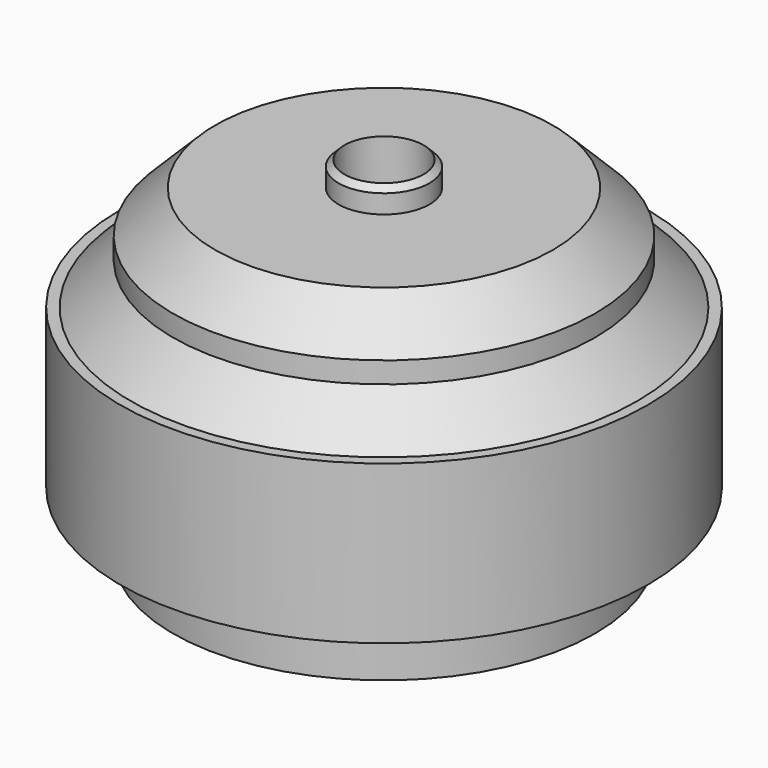
from build123d import *

# Parameters (mm, degrees)
F2_R     = 4.7625
F3_DEPTH = 9.525
F6_D     = 3.175
F6_DEPTH = 22.225
F6_START = 0.6225488
F6_TIP   = 0.9538662327
F7_SIZE  = 5.08


# Not quite as in the source:
# - a fillet or chamfer that OpenCascade refuses, or shapes differently, is made with other operations: its cross-section is extruded or revolved along the edge and cut away or added


with BuildPart() as f1:
    # F0 (on Front) → F1 (revolve)
    with BuildSketch(Plane.XZ):
        Polygon((5.470779, 56.2707707286), (0, 56.2707707286), (0, 0), (25.409779, 9.9646151066), (25.409779, 17.1938474178), (31.759779, 17.1938474178), (31.759779, 36.2438474178), (25.409779, 36.2438474178), (25.409779, 48.9438474178), (5.470779, 48.9438474178), align=None)
    revolve(axis=Axis((0, 0, 28.1353853643), (0, 0, -1)))

    # F2 (on face) → F3 (cut)
    with BuildSketch(Plane.XY.offset(56.2707707286)):
        Circle(F2_R)
    extrude(amount=-F3_DEPTH, mode=Mode.SUBTRACT)

    # F4: chamfer of 5.08 on 1 edges, made by hand

    # F4_s1 → F4_t2 (revolve, cut)
    with BuildSketch(Plane.XZ):
        Polygon((0.390779, 56.2707707286), (5.470779, 51.1907707286), (5.470779, 56.2707707286), align=None)
    revolve(axis=Axis((0, 0, 56.2707707286), (0, 0, -1)), mode=Mode.SUBTRACT)

    # F6
    # its depths count from where the whole tool has entered the part; down to there all is cleared
    with Locations(Plane(origin=(0, 0, 0), x_dir=(1, 0, 0), z_dir=(0, 0, -1)).offset(-F6_START)):
        with Locations((0, 0)):
            Hole(F6_D / 2, depth=F6_DEPTH)
            with Locations((0, 0, -(F6_DEPTH + F6_TIP / 2))):  # 118° drill point
                Cone(0, F6_D / 2, F6_TIP, mode=Mode.SUBTRACT)

    # F7
    f7_edges = [f1.edges().sort_by_distance(p)[0] for p in [
        (-25.409779, 0, 36.243847),
        (-25.409779, 0, 48.943847),
        (25.409779, 0, 42.593847),
    ]]
    chamfer(f7_edges, length=F7_SIZE)


solid = f1.part
